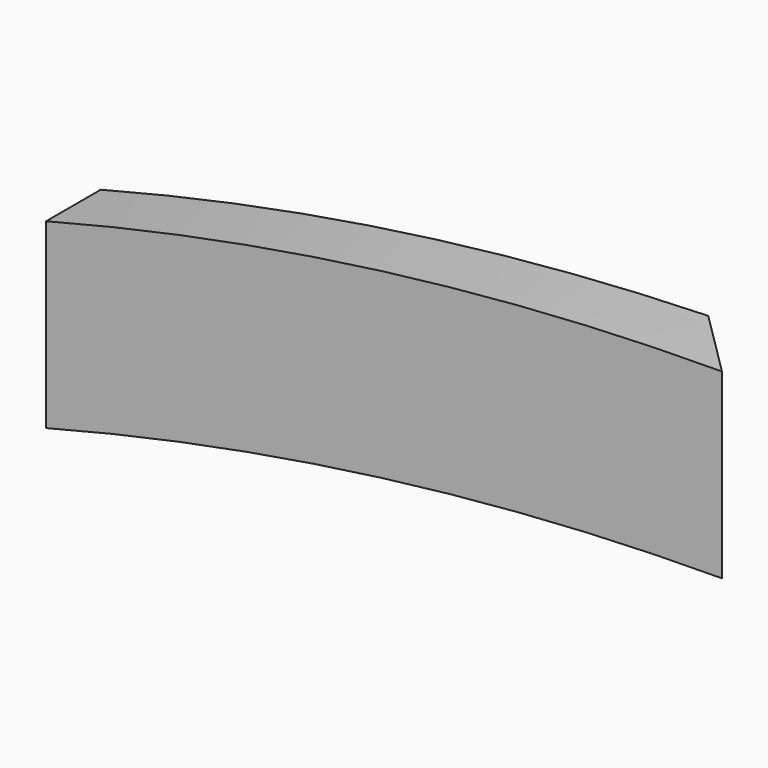
from build123d import *

# Parameters (mm, degrees)
F1_DEPTH    = 7.5
F2_T1_DEPTH = 61.1469278075


# Not quite as in the source:
# - a fillet or chamfer that OpenCascade refuses, or shapes differently, is made with other operations: its cross-section is extruded or revolved along the edge and cut away or added
# - a feature names something its author has since deleted; it is built from what else it names


with BuildPart() as f1:
    # F0 (on Front) → F1 (new body)
    with BuildSketch(Plane.XZ):
        with BuildLine():
            Line((-74.7255906463, 20), (-74.7255906463, 0))
            ThreePointArc((-74.7255906463, 0), (-37.6697049266, 7.1922767475), (0, 9.613194347))
            Line((0, 9.613194347), (0, 29.613194347))
            ThreePointArc((0, 29.613194347), (-37.6697049266, 27.1922767475), (-74.7255906463, 20))
        make_face()
    extrude(amount=F1_DEPTH)

    # F2: chamfer of 8 on 1 edges, made by hand

    # F2_s2 → F2_t1 (cut)
    with BuildSketch(Plane.XY.offset(-10.9602695567)):
        Polygon((0, -8), (-8, 0), (0, 0), align=None)
    extrude(amount=F2_T1_DEPTH, mode=Mode.SUBTRACT)


solid = f1.part
